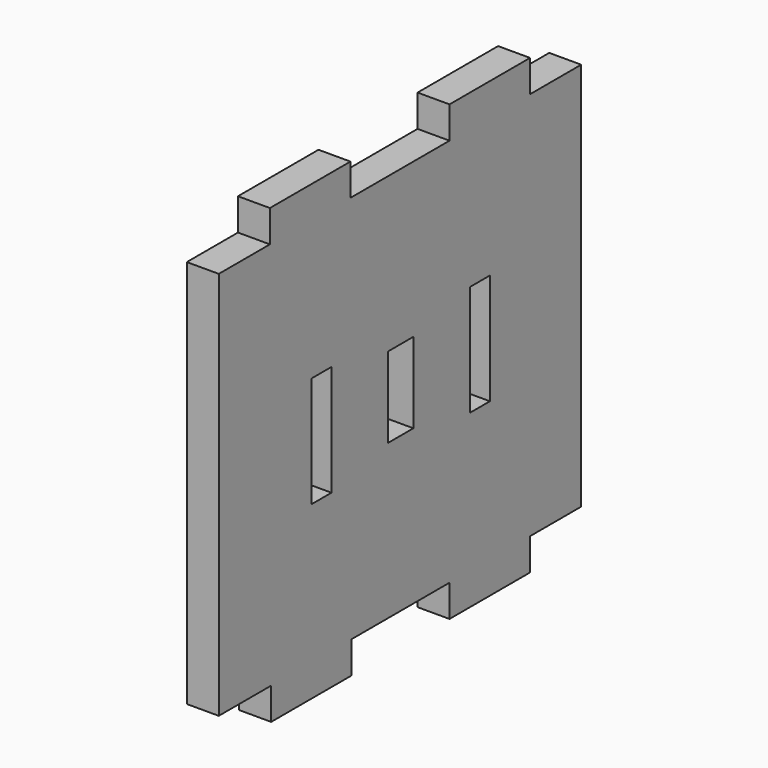
from build123d import *

# Parameters (mm, degrees)
F1_DEPTH = 3.175


# Not quite as in the source:
# - a length typed as a fraction of an inch, garbled in the dataset ("3 / 203.2 mm" for 3/8 in), is restored


with BuildPart() as f1:
    # F0 (on Right) → F1 (new body)
    with BuildSketch(Plane.YZ):
        Polygon((16.0724163434, -25.675), (16.0724163434, -22.5), (22.4224163434, -22.5), (22.4224163434, 16.15), (16.0724163434, 16.15), (16.0724163434, 19.325), (6.0724163434, 19.325), (6.0724163434, 16.15), (-6.2275836566, 16.15), (-6.2275836566, 19.325), (-16.2275836566, 19.325), (-16.2275836566, 16.15), (-19.4025836566, 16.15), (-19.325, -22.5), (-16.0724163434, -22.5), (-16.0724163434, -25.675), (-6.0724163434, -25.675), (-6.0724163434, -24.0875), (-6.0724163434, -22.5), (6.0724163434, -22.5), (6.0724163434, -24.0875), (6.0724163434, -25.675), align=None)
        Polygon((-8.5875, 2.325), (-8.5875, -3.175), (-8.5875, -8.675), (-11.0875, -8.675), (-11.0875, 2.325), align=None, mode=Mode.SUBTRACT)
        Polygon((1.5875, -3.175), (1.5875, -7.175), (-1.5875, -7.175), (-1.5875, -3.175), (-1.5875, 0.825), (1.5875, 0.825), align=None, mode=Mode.SUBTRACT)
        Polygon((8.5875, -8.675), (8.5875, -3.175), (8.5875, 2.325), (11.0875, 2.325), (11.0875, -8.675), align=None, mode=Mode.SUBTRACT)
        Polygon((-22.5775836566, -22.5), (-19.325, -22.5), (-19.4025836566, 16.15), (-22.5775836566, 16.15), align=None)
    extrude(amount=F1_DEPTH)


solid = f1.part
